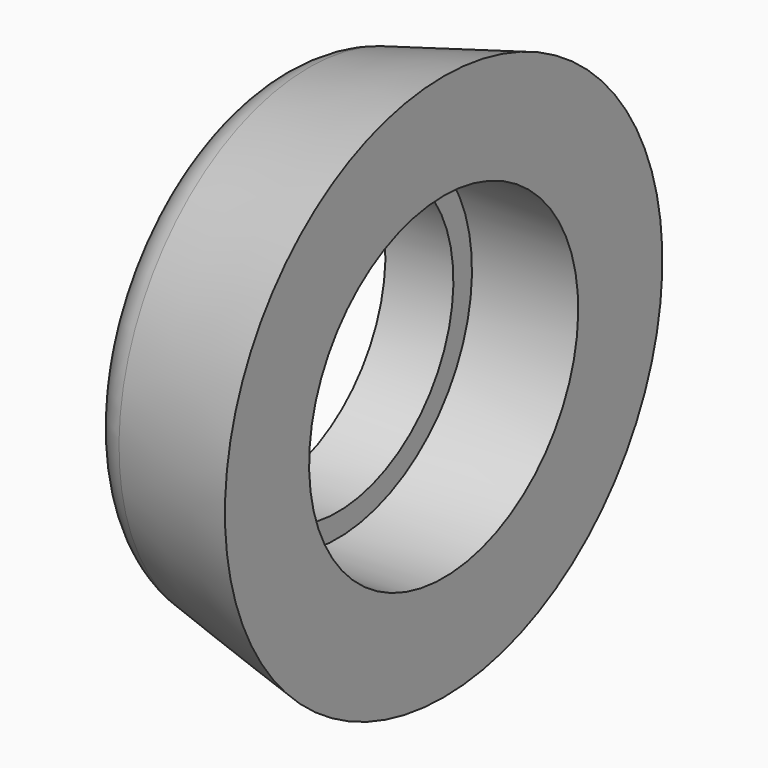
from build123d import *


# Not quite as in the source:
# - a feature names something its author has since deleted; it is built from what else it names


with BuildPart() as f1:
    # F0 (on Front) → F1 (revolve)
    with BuildSketch(Plane.XZ):
        with BuildLine():
            Line((0, 7.540625), (0, 12.2555))
            Line((0, 12.2555), (-6.0455628512, 10.6355963162))
            ThreePointArc((-6.0455628512, 10.6355963162), (-7.3184226416, 9.7850985952), (-7.8105, 8.3354854424))
            Line((-7.8105, 8.3354854424), (-7.8105, 6.49986))
            Line((-7.8105, 6.49986), (-4.7625, 6.49986))
            Line((-4.7625, 6.49986), (-4.7625, 7.540625))
            Line((-4.7625, 7.540625), (0, 7.540625))
        make_face()
    revolve(axis=Axis((5.2561350167, 0, 0), (1, 0, 0)))


solid = f1.part
